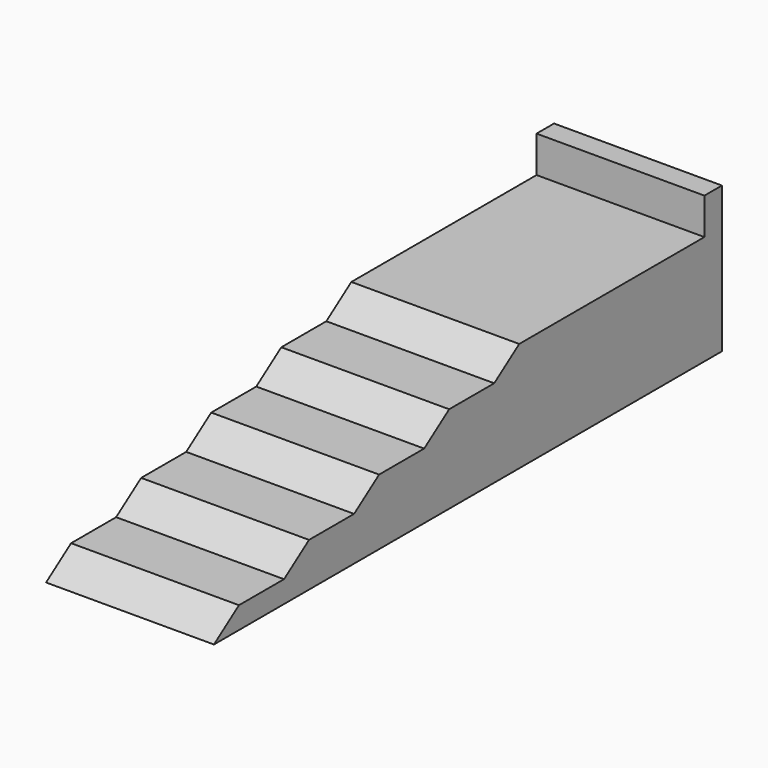
from build123d import *

# Parameters (mm, degrees)
F0_W        = 1066.8
F0_H        = 38.1
F1_DEPTH    = 292.1
F2_W        = 914.4
F2_H        = 38.1
F3_DEPTH    = 292.1
F4_W        = 762
F4_H        = 38.1
F5_DEPTH    = 292.1
F6_W        = 609.6
F6_H        = 38.1
F7_DEPTH    = 292.1
F8_W        = 457.2
F8_H        = 38.1
F9_DEPTH    = 292.1
F10_SIZE2   = 54.412429
F10_SIZE    = 38.09999
F10_2_SIZE2 = 54.412429
F10_2_SIZE  = 38.09999
F10_3_SIZE2 = 54.412429
F10_3_SIZE  = 38.09999
F10_4_SIZE2 = 54.412429
F10_4_SIZE  = 38.09999
F10_5_SIZE2 = 54.412429
F10_5_SIZE  = 38.09999
F11_W       = 292.1000000001
F11_H       = 38.1
F12_DEPTH   = 254


# Not quite as in the source:
# - a fillet or chamfer is up to 0.001 mm smaller than in the source, because OpenCascade refuses the exact size


with BuildPart() as f1:
    # F0 (on Right) → F1 (new body)
    with BuildSketch(Plane.YZ):
        with Locations((533.4, 19.05)):
            Rectangle(F0_W, F0_H)
    extrude(amount=F1_DEPTH)

    # F2 (on Right) → F3 (join, through all)
    with BuildSketch(Plane.YZ):
        with Locations((609.6, 57.15)):
            Rectangle(F2_W, F2_H)
    extrude(amount=F3_DEPTH)

    # F4 (on Right) → F5 (join, through all)
    with BuildSketch(Plane.YZ):
        with Locations((685.8, 95.25)):
            Rectangle(F4_W, F4_H)
    extrude(amount=F5_DEPTH)

    # F6 (on Right) → F7 (join, through all)
    with BuildSketch(Plane.YZ):
        with Locations((762, 133.35)):
            Rectangle(F6_W, F6_H)
    extrude(amount=F7_DEPTH)

    # F8 (on Right) → F9 (join, through all)
    with BuildSketch(Plane.YZ):
        with Locations((838.2, 171.45)):
            Rectangle(F8_W, F8_H)
    extrude(amount=F9_DEPTH)

    # F10 (size 38.1 and 54.4124390569 in the source; OpenCascade refuses exactly that, so slightly less here)
    f10_edges = [f1.edges().sort_by_distance(p)[0] for p in [
        (146.05, 0, 38.1),
    ]]
    f10_side = f1.faces().sort_by_distance((146.05, 0, 19.05))[0]
    chamfer(f10_edges, length=F10_SIZE, length2=F10_SIZE2, reference=f10_side)

    # F10#2 (size 38.1 and 54.4124390569 in the source; OpenCascade refuses exactly that, so slightly less here)
    f10_2_edges = [f1.edges().sort_by_distance(p)[0] for p in [
        (146.05, 152.4, 76.2),
    ]]
    f10_2_side = f1.faces().sort_by_distance((146.05, 152.4, 57.15))[0]
    chamfer(f10_2_edges, length=F10_2_SIZE, length2=F10_2_SIZE2, reference=f10_2_side)

    # F10#3 (size 38.1 and 54.4124390569 in the source; OpenCascade refuses exactly that, so slightly less here)
    f10_3_edges = [f1.edges().sort_by_distance(p)[0] for p in [
        (146.05, 304.8, 114.3),
    ]]
    f10_3_side = f1.faces().sort_by_distance((146.05, 304.8, 95.25))[0]
    chamfer(f10_3_edges, length=F10_3_SIZE, length2=F10_3_SIZE2, reference=f10_3_side)

    # F10#4 (size 38.1 and 54.4124390569 in the source; OpenCascade refuses exactly that, so slightly less here)
    f10_4_edges = [f1.edges().sort_by_distance(p)[0] for p in [
        (146.05, 457.2, 152.4),
    ]]
    f10_4_side = f1.faces().sort_by_distance((146.05, 457.2, 133.35))[0]
    chamfer(f10_4_edges, length=F10_4_SIZE, length2=F10_4_SIZE2, reference=f10_4_side)

    # F10#5 (size 38.1 and 54.4124390569 in the source; OpenCascade refuses exactly that, so slightly less here)
    f10_5_edges = [f1.edges().sort_by_distance(p)[0] for p in [
        (146.05, 609.6, 190.5),
    ]]
    f10_5_side = f1.faces().sort_by_distance((146.05, 609.6, 171.45))[0]
    chamfer(f10_5_edges, length=F10_5_SIZE, length2=F10_5_SIZE2, reference=f10_5_side)

    # F11 (on Top) → F12 (join)
    with BuildSketch(Plane.XY):
        with Locations((146.0500000001, 1085.85)):
            Rectangle(F11_W, F11_H)
    extrude(amount=F12_DEPTH)


solid = f1.part
